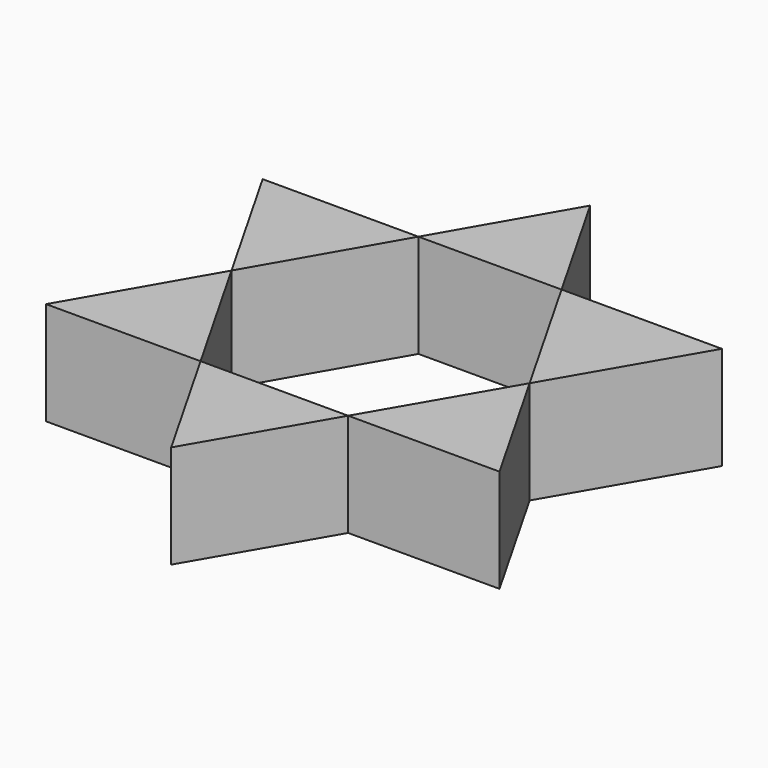
from build123d import *

# Parameters (mm, degrees)
F5_DEPTH = 10


# Not quite as in the source:
# - the program builds the solid bodies; features that only make, move or delete a surface that nothing else refers to are left out


with BuildPart() as f5:
    # F1 (on Top) → F5 (new body)
    with BuildSketch(Plane.XY):
        Polygon((-6.9625685365, 13.063011691), (-22.0539048314, 13.063011691), (-14.5391420015, -0.104448899), align=None)
    extrude(amount=F5_DEPTH)


with BuildPart() as f5b:
    # F1 (on Top) → F5, piece 2 (new body)
    with BuildSketch(Plane.XY):
        Polygon((0, 25.1633822918), (-6.9625685365, 13.063011691), (6.9057670306, 13.063011691), align=None)
    extrude(amount=F5_DEPTH)


with BuildPart() as f5c:
    # F1 (on Top) → F5, piece 3 (new body)
    with BuildSketch(Plane.XY):
        Polygon((22.4442388862, 13.063011691), (6.9057670306, 13.063011691), (14.6068518602, -0.4309246167), align=None)
    extrude(amount=F5_DEPTH)


with BuildPart() as f5d:
    # F1 (on Top) → F5, piece 4 (new body)
    with BuildSketch(Plane.XY):
        Polygon((21.8739863143, -13.1644876968), (14.6068518602, -0.4309246167), (7.2110957366, -13.1644876968), align=None)
    extrude(amount=F5_DEPTH)


with BuildPart() as f5e:
    # F1 (on Top) → F5, piece 5 (new body)
    with BuildSketch(Plane.XY):
        Polygon((7.2110957366, -13.1644876968), (-7.0856855477, -13.1644876968), (0, -25.5801137537), align=None)
    extrude(amount=F5_DEPTH)


with BuildPart() as f5f:
    # F1 (on Top) → F5, piece 6 (new body)
    with BuildSketch(Plane.XY):
        Polygon((-7.0856855477, -13.1644876968), (-14.5391420015, -0.104448899), (-22.0539048314, -13.1644876968), align=None)
    extrude(amount=F5_DEPTH)


solid = Compound([f5.part, f5b.part, f5c.part, f5d.part, f5e.part, f5f.part])
